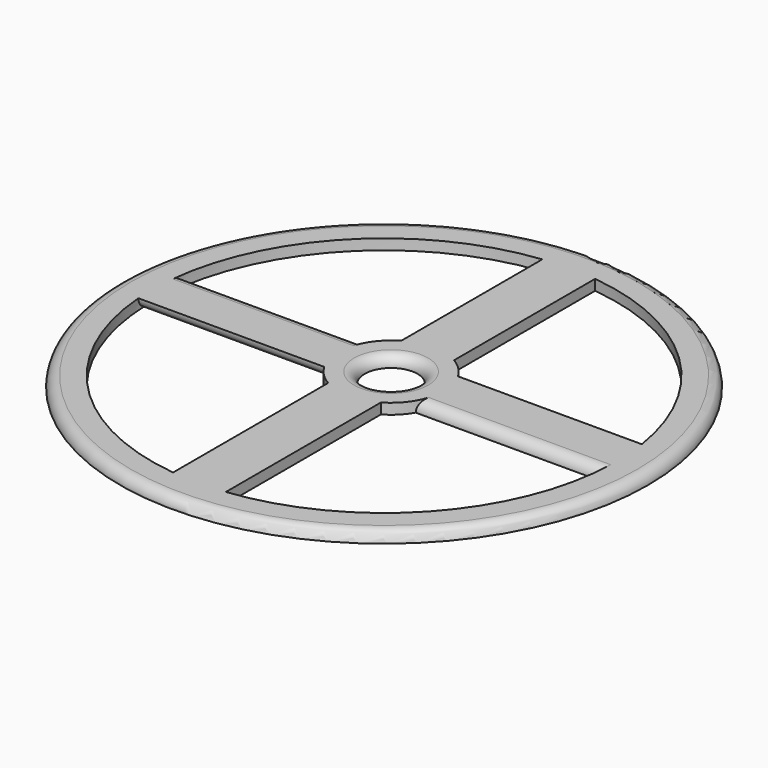
from build123d import *

# Parameters (mm, degrees)
F0_R     = 50
F0_R_2   = 5
F1_DEPTH = 2
F2_R     = 1.99999


# Not quite as in the source:
# - a fillet or chamfer is up to 0.001 mm smaller than in the source, because OpenCascade refuses the exact size


with BuildPart() as f1:
    # F0 (on Top) → F1 (new body)
    with BuildSketch(Plane.XY):
        with Locations((0, -1.6630436294)):
            Circle(F0_R)
        with BuildLine():
            ThreePointArc((-5, -45.3780296182), (-31.6977238962, -32.1795031194), (-43.873280276, -5))
            Line((-43.873280276, -5), (-8.6602540378, -5))
            ThreePointArc((-8.6602540378, -5), (-7.0710678119, -7.0710678119), (-5, -8.6602540378))
            Line((-5, -8.6602540378), (-5, -45.3780296182))
        make_face(mode=Mode.SUBTRACT)
        with BuildLine():
            ThreePointArc((5, -8.6602540378), (7.0710678119, -7.0710678119), (8.6602540378, -5))
            Line((8.6602540378, -5), (43.873280276, -5))
            ThreePointArc((43.873280276, -5), (31.6977238962, -32.1795031194), (5, -45.3780296182))
            Line((5, -45.3780296182), (5, -8.6602540378))
        make_face(mode=Mode.SUBTRACT)
        with BuildLine():
            ThreePointArc((-43.4925723497, 5), (-30.513832952, 30.0372087131), (-5, 42.0519423594))
            Line((-5, 42.0519423594), (-5, 8.6602540378))
            ThreePointArc((-5, 8.6602540378), (-7.0710678119, 7.0710678119), (-8.6602540378, 5))
            Line((-8.6602540378, 5), (-43.4925723497, 5))
        make_face(mode=Mode.SUBTRACT)
        Circle(F0_R_2, mode=Mode.SUBTRACT)
        with BuildLine():
            Line((43.4925723497, 5), (8.6602540378, 5))
            ThreePointArc((8.6602540378, 5), (7.0710678119, 7.0710678119), (5, 8.6602540378))
            Line((5, 8.6602540378), (5, 42.0519423594))
            ThreePointArc((5, 42.0519423594), (30.513832952, 30.0372087131), (43.4925723497, 5))
        make_face(mode=Mode.SUBTRACT)
    extrude(amount=F1_DEPTH)

    # F2 (radius 2 in the source; OpenCascade refuses exactly that, so slightly less here)
    f2_edges = [f1.edges().sort_by_distance(p)[0] for p in [
        (-50, -1.663044, 2),
        (26.076413, 5, 0),
        (-26.266767, -5, 0),
        (-26.076413, 5, 2),
        (26.266767, -5, 2),
        (-5, 0, 2),
    ]]
    fillet(f2_edges, radius=F2_R)


solid = f1.part
